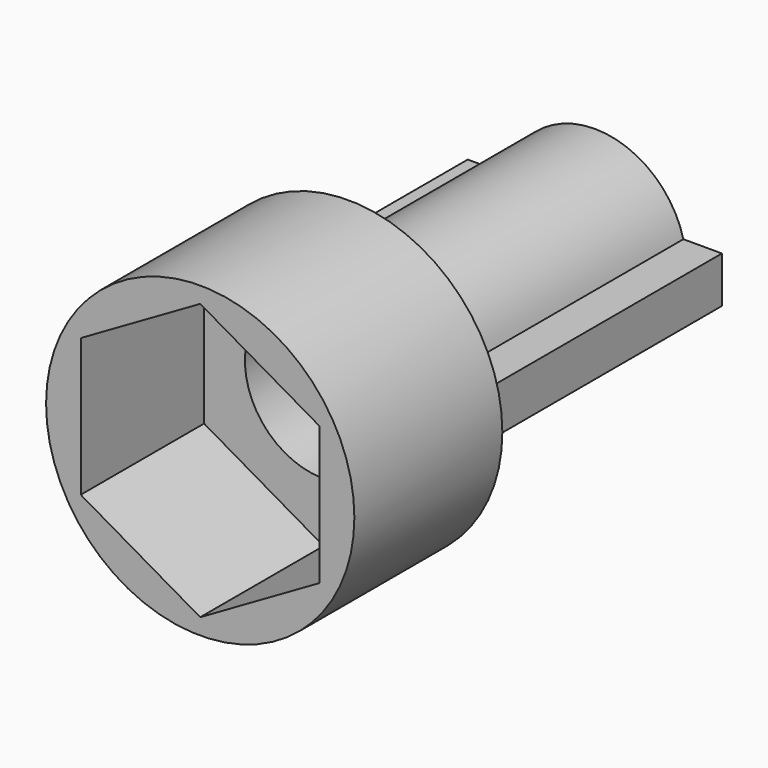
from build123d import *

# Parameters (mm, degrees)
F0_R     = 12.7
F0_W     = 0.6285263425
F0_H     = 3.81
F1_DEPTH = 12.7
F2_DEPTH = 2.54
F0_R_2   = 6.477
F3_DEPTH = 27.94


# Not quite as in the source:
# - a feature names something its author has since deleted; it is built from what else it names


with BuildPart() as f1:
    # F0 (on Front) → F1 (new body)
    with BuildSketch(Plane.XZ):
        Circle(F0_R)
        Polygon((9.8425, 5.6825700245), (9.8425, 1.905), (10.4710263425, 1.905), (10.4710263425, -1.905), (9.8425, -1.905), (9.8425, -5.6825700245), (0, -11.365140049), (-9.8425, -5.6825700245), (-9.8425, -1.905), (-10.4710263425, -1.905), (-10.4710263425, 1.905), (-9.8425, 1.905), (-9.8425, 5.6825700245), (0, 11.365140049), align=None, mode=Mode.SUBTRACT)
        with Locations((10.1567631713, 0)):
            Rectangle(F0_W, F0_H)
        with Locations((-10.1567631713, 0)):
            Rectangle(F0_W, F0_H)
    extrude(amount=F1_DEPTH)

    # F0 (on Front) → F2 (join)
    with BuildSketch(Plane.XZ):
        Circle(F0_R)
        Polygon((9.8425, 5.6825700245), (9.8425, 1.905), (10.4710263425, 1.905), (10.4710263425, -1.905), (9.8425, -1.905), (9.8425, -5.6825700245), (0, -11.365140049), (-9.8425, -5.6825700245), (-9.8425, -1.905), (-10.4710263425, -1.905), (-10.4710263425, 1.905), (-9.8425, 1.905), (-9.8425, 5.6825700245), (0, 11.365140049), align=None, mode=Mode.SUBTRACT)
        with BuildLine():
            ThreePointArc((-7.2960263425, 1.905), (0, 7.540625), (7.2960263425, 1.905))
            Line((7.2960263425, 1.905), (9.8425, 1.905))
            Line((9.8425, 1.905), (9.8425, 5.6825700245))
            Line((9.8425, 5.6825700245), (0, 11.365140049))
            Line((0, 11.365140049), (-9.8425, 5.6825700245))
            Line((-9.8425, 5.6825700245), (-9.8425, 1.905))
            Line((-9.8425, 1.905), (-7.2960263425, 1.905))
        make_face()
        with BuildLine():
            Line((9.8425, -1.905), (7.2960263425, -1.905))
            ThreePointArc((7.2960263425, -1.905), (0, -7.540625), (-7.2960263425, -1.905))
            Line((-7.2960263425, -1.905), (-9.8425, -1.905))
            Line((-9.8425, -1.905), (-9.8425, -5.6825700245))
            Line((-9.8425, -5.6825700245), (0, -11.365140049))
            Line((0, -11.365140049), (9.8425, -5.6825700245))
            Line((9.8425, -5.6825700245), (9.8425, -1.905))
        make_face()
    extrude(amount=-F2_DEPTH)

    # F0 (on Front) → F3 (join)
    with BuildSketch(Plane.XZ):
        with BuildLine():
            ThreePointArc((7.2960263425, 1.905), (7.4792253619, 0.9603194134), (7.540625, 0))
            ThreePointArc((7.540625, 0), (7.4792253619, -0.9603194134), (7.2960263425, -1.905))
            Line((7.2960263425, -1.905), (9.8425, -1.905))
            Line((9.8425, -1.905), (9.8425, 1.905))
            Line((9.8425, 1.905), (7.2960263425, 1.905))
        make_face()
        with BuildLine():
            ThreePointArc((7.2960263425, -1.905), (7.4792253619, -0.9603194134), (7.540625, 0))
            ThreePointArc((7.540625, 0), (7.4792253619, 0.9603194134), (7.2960263425, 1.905))
            Line((7.2960263425, 1.905), (7.2960263425, -1.905))
        make_face()
        with BuildLine():
            Line((7.2960263425, -1.905), (7.2960263425, 1.905))
            ThreePointArc((7.2960263425, 1.905), (0, 7.540625), (-7.2960263425, 1.905))
            Line((-7.2960263425, 1.905), (-7.2960263425, -1.905))
            ThreePointArc((-7.2960263425, -1.905), (0, -7.540625), (7.2960263425, -1.905))
        make_face()
        Circle(F0_R_2, mode=Mode.SUBTRACT)
        with BuildLine():
            Line((-7.2960263425, -1.905), (-7.2960263425, 1.905))
            ThreePointArc((-7.2960263425, 1.905), (-7.540625, 0), (-7.2960263425, -1.905))
        make_face()
        with BuildLine():
            ThreePointArc((-7.2960263425, -1.905), (-7.540625, 0), (-7.2960263425, 1.905))
            Line((-7.2960263425, 1.905), (-9.8425, 1.905))
            Line((-9.8425, 1.905), (-9.8425, -1.905))
            Line((-9.8425, -1.905), (-7.2960263425, -1.905))
        make_face()
        with Locations((10.1567631713, 0)):
            Rectangle(F0_W, F0_H)
        with Locations((-10.1567631713, 0)):
            Rectangle(F0_W, F0_H)
    extrude(amount=-F3_DEPTH)


solid = f1.part
